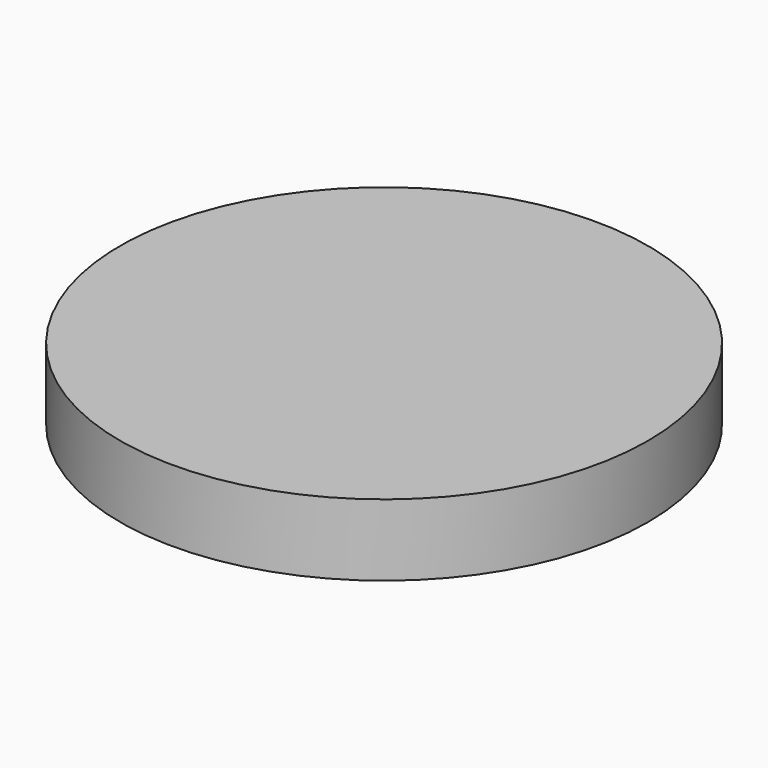
from build123d import *

# Parameters (mm, degrees)
F3_R     = 75.8455740266
F4_DEPTH = 20.5738395452


# Not quite as in the source:
# - the program builds the solid bodies; features that only make, move or delete a surface that nothing else refers to are left out


with BuildPart() as f4:
    # F3 (on Top) → F4 (new body)
    with BuildSketch(Plane.XY):
        Circle(F3_R)
    extrude(amount=-F4_DEPTH)


solid = f4.part
